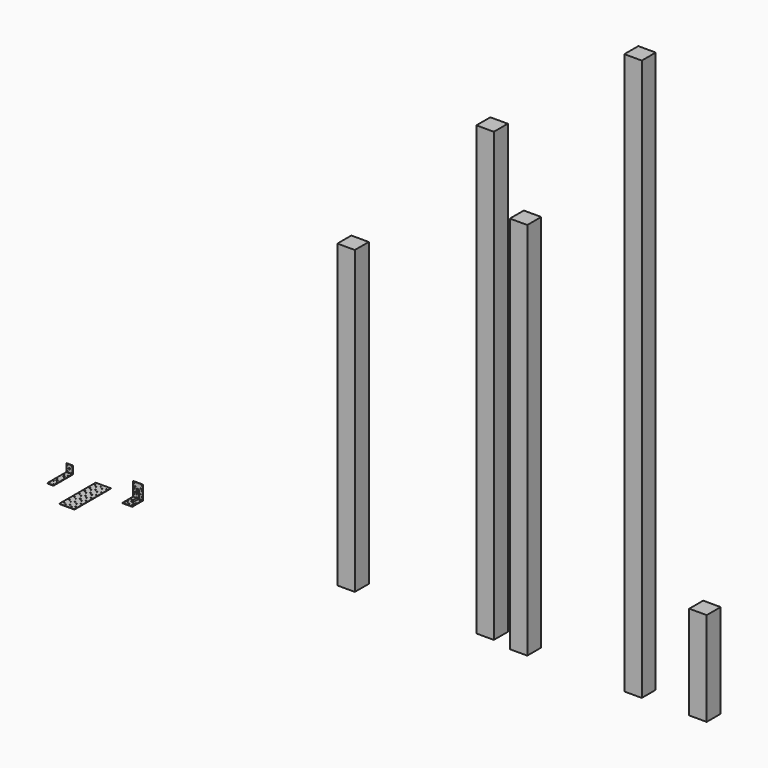
from build123d import *

# Parameters (mm, degrees)
F0_W      = 115
F0_H      = 115
F1_DEPTH  = 1985
F2_W      = 115
F2_H      = 115
F3_DEPTH  = 2950
F4_W      = 115
F4_H      = 115
F5_DEPTH  = 2500
F6_W      = 115
F6_H      = 115
F7_DEPTH  = 3700
F8_W      = 115
F8_H      = 115
F9_DEPTH  = 620
F10_W     = 65
F10_H     = 90
F10_R     = 2.5
F10_R_2   = 4
F11_DEPTH = 2.5
F12_W     = 65
F12_H     = 2.5
F13_DEPTH = 90
F14_W     = 7
F14_H     = 49.849742502
F15_DEPTH = 5
F16_W     = 14
F16_H     = 50
F17_DEPTH = 5
F18_F1_R  = 5
F18_F2_R  = 4.9999
F16_R     = 2.5
F19_DEPTH = 25
F20_W     = 100
F20_H     = 300
F20_R     = 3
F21_DEPTH = 2
F22_W     = 40
F22_H     = 160
F23_DEPTH = 3
F24_W     = 40
F24_H     = 3
F25_DEPTH = 50
F26_R     = 5
F26_R_2   = 2.5
F27_DEPTH = 25
F28_R     = 2
F29_R     = 2.5
F29_R_2   = 5
F30_DEPTH = 25


# Not quite as in the source:
# - a fillet or chamfer is up to 0.001 mm smaller than in the source, because OpenCascade refuses the exact size


with BuildPart() as f1:
    # F0 (on Top) → F1 (new body)
    with BuildSketch(Plane.XY):
        with Locations((-57.5, -57.5)):
            Rectangle(F0_W, F0_H)
    extrude(amount=F1_DEPTH)


with BuildPart() as f3:
    # F2 (on Top) → F3 (new body)
    with BuildSketch(Plane.XY):
        with Locations((835.767865181, -28.2673428646)):
            Rectangle(F2_W, F2_H)
    extrude(amount=F3_DEPTH)


with BuildPart() as f5:
    # F4 (on Top) → F5 (new body)
    with BuildSketch(Plane.XY):
        with Locations((1079.8359951153, -57.5)):
            Rectangle(F4_W, F4_H)
    extrude(amount=F5_DEPTH)


with BuildPart() as f7:
    # F6 (on Top) → F7 (new body)
    with BuildSketch(Plane.XY):
        with Locations((1834.8243838341, -57.5)):
            Rectangle(F6_W, F6_H)
    extrude(amount=F7_DEPTH)


with BuildPart() as f9:
    # F8 (on Top) → F9 (new body)
    with BuildSketch(Plane.XY):
        with Locations((2262.808675766, -57.5)):
            Rectangle(F8_W, F8_H)
    extrude(amount=F9_DEPTH)


with BuildPart() as f11:
    # F10 (on Top) → F11 (new body)
    with BuildSketch(Plane.XY):
        with Locations((-1520.1824146039, -45)):
            Rectangle(F10_W, F10_H)
        with Locations((-1544.6824146039, -81.6684067249)):
            Circle(F10_R, mode=Mode.SUBTRACT)
        with Locations((-1539.6824146039, -63.6286884546)):
            Circle(F10_R, mode=Mode.SUBTRACT)
        with Locations((-1544.6824146039, -50.4504516721)):
            Circle(F10_R, mode=Mode.SUBTRACT)
        with Locations((-1520.1824146039, -77.8877660632)):
            Circle(F10_R_2, mode=Mode.SUBTRACT)
        with Locations((-1495.6824146039, -81.6684067249)):
            Circle(F10_R, mode=Mode.SUBTRACT)
        with Locations((-1500.6824146039, -63.6286884546)):
            Circle(F10_R, mode=Mode.SUBTRACT)
        with Locations((-1495.6824146039, -50.4504516721)):
            Circle(F10_R, mode=Mode.SUBTRACT)
        with Locations((-1539.6824146039, -30.1858838648)):
            Circle(F10_R, mode=Mode.SUBTRACT)
        with Locations((-1544.6824146039, -15.9201901406)):
            Circle(F10_R, mode=Mode.SUBTRACT)
        with Locations((-1500.6824146039, -30.1858838648)):
            Circle(F10_R, mode=Mode.SUBTRACT)
        with Locations((-1495.6824146039, -15.9201901406)):
            Circle(F10_R, mode=Mode.SUBTRACT)
    extrude(amount=F11_DEPTH)

    # F12 (on face) → F13 (join)
    with BuildSketch(Plane.XY.offset(2.5)):
        with Locations((-1520.1824146039, -1.25)):
            Rectangle(F12_W, F12_H)
    extrude(amount=F13_DEPTH)

    # F14 (on face) → F15 (join)
    with BuildSketch(Plane.XY.offset(2.5)):
        with Locations((-1516.6824146039, -27.424871251)):
            Rectangle(F14_W, F14_H)
        with Locations((-1523.6824146039, -27.424871251)):
            Rectangle(F14_W, F14_H)
    extrude(amount=F15_DEPTH)

    # F16 (on face) → F17 (join)
    with BuildSketch(Plane.XZ.offset(2.5)):
        with Locations((-1520.1824146039, 32.5)):
            Rectangle(F16_W, F16_H)
    extrude(amount=F17_DEPTH)

    # F18: fillet of radius 5 on 5 edges, made by hand

    # F18_f1
    f18_f1_edges = [f11.edges().sort_by_distance(p)[0] for p in [
        (-1520.1824146039, -7.5, 7.5),
    ]]
    fillet(f18_f1_edges, radius=F18_F1_R)

    # F18_f2 (radius 5 in the source; OpenCascade refuses exactly that, so slightly less here)
    f18_f2_edges = [f11.edges().sort_by_distance(p)[0] for p in [
        (-1527.1824146039, -32.424871251, 7.5),
        (-1513.1824146039, -7.5, 35),
        (-1520.1824146039, -52.349742502, 7.5),
        (-1520.1824146039, -7.5, 57.5),
        (-1513.1824146039, -8.9644660941, 8.9644660941),
        (-1527.1824146039, -8.9644660941, 8.9644660941),
    ]]
    fillet(f18_f2_edges, radius=F18_F2_R)

    # F16 (on face) → F19 (cut)
    with BuildSketch(Plane.XZ.offset(2.5)):
        with Locations((-1544.6824146039, 18.7368597835)):
            Circle(F16_R)
        with Locations((-1539.6824146039, 33.0025535077)):
            Circle(F16_R)
        with Locations((-1544.6824146039, 53.267121315)):
            Circle(F16_R)
        with Locations((-1539.6824146039, 66.4453580976)):
            Circle(F16_R)
        with Locations((-1544.6824146039, 84.4850763679)):
            Circle(F16_R)
        with Locations((-1495.6824146039, 84.4850763679)):
            Circle(F16_R)
        with Locations((-1500.6824146039, 66.4453580976)):
            Circle(F16_R)
        with Locations((-1495.6824146039, 53.267121315)):
            Circle(F16_R)
        with Locations((-1500.6824146039, 33.0025535077)):
            Circle(F16_R)
        with Locations((-1495.6824146039, 18.7368597835)):
            Circle(F16_R)
    extrude(amount=-F19_DEPTH, mode=Mode.SUBTRACT)


with BuildPart() as f21:
    # F20 (on Top) → F21 (new body)
    with BuildSketch(Plane.XY):
        with Locations((-1750.8230004184, -150)):
            Rectangle(F20_W, F20_H)
        with Locations((-1788.8230004184, -273.6264169216)):
            Circle(F20_R, mode=Mode.SUBTRACT)
        with Locations((-1788.8230004184, -231.6264169216)):
            Circle(F20_R, mode=Mode.SUBTRACT)
        with Locations((-1769.8230004184, -286.8777215481)):
            Circle(F20_R, mode=Mode.SUBTRACT)
        with Locations((-1750.8230004184, -273.6264169216)):
            Circle(F20_R, mode=Mode.SUBTRACT)
        with Locations((-1769.8230004184, -244.8777215481)):
            Circle(F20_R, mode=Mode.SUBTRACT)
        with Locations((-1750.8230004184, -231.6264169216)):
            Circle(F20_R, mode=Mode.SUBTRACT)
        with Locations((-1788.8230004184, -189.6264169216)):
            Circle(F20_R, mode=Mode.SUBTRACT)
        with Locations((-1769.8230004184, -202.8777215481)):
            Circle(F20_R, mode=Mode.SUBTRACT)
        with Locations((-1750.8230004184, -189.6264169216)):
            Circle(F20_R, mode=Mode.SUBTRACT)
        with Locations((-1769.8230004184, -160.8777215481)):
            Circle(F20_R, mode=Mode.SUBTRACT)
        with Locations((-1731.8230004184, -286.8777215481)):
            Circle(F20_R, mode=Mode.SUBTRACT)
        with Locations((-1731.8230004184, -244.8777215481)):
            Circle(F20_R, mode=Mode.SUBTRACT)
        with Locations((-1712.8230004184, -273.6264169216)):
            Circle(F20_R, mode=Mode.SUBTRACT)
        with Locations((-1712.8230004184, -231.6264169216)):
            Circle(F20_R, mode=Mode.SUBTRACT)
        with Locations((-1731.8230004184, -202.8777215481)):
            Circle(F20_R, mode=Mode.SUBTRACT)
        with Locations((-1731.8230004184, -160.8777215481)):
            Circle(F20_R, mode=Mode.SUBTRACT)
        with Locations((-1712.8230004184, -189.6264169216)):
            Circle(F20_R, mode=Mode.SUBTRACT)
        with Locations((-1788.8230004184, -147.6264169216)):
            Circle(F20_R, mode=Mode.SUBTRACT)
        with Locations((-1788.8230004184, -105.6264169216)):
            Circle(F20_R, mode=Mode.SUBTRACT)
        with Locations((-1769.8230004184, -118.8777215481)):
            Circle(F20_R, mode=Mode.SUBTRACT)
        with Locations((-1750.8230004184, -147.6264169216)):
            Circle(F20_R, mode=Mode.SUBTRACT)
        with Locations((-1769.8230004184, -76.8777215481)):
            Circle(F20_R, mode=Mode.SUBTRACT)
        with Locations((-1750.8230004184, -105.6264169216)):
            Circle(F20_R, mode=Mode.SUBTRACT)
        with Locations((-1788.8230004184, -63.6264169216)):
            Circle(F20_R, mode=Mode.SUBTRACT)
        with Locations((-1788.8230004184, -21.6264169216)):
            Circle(F20_R, mode=Mode.SUBTRACT)
        with Locations((-1750.8230004184, -63.6264169216)):
            Circle(F20_R, mode=Mode.SUBTRACT)
        with Locations((-1769.8230004184, -34.8777215481)):
            Circle(F20_R, mode=Mode.SUBTRACT)
        with Locations((-1750.8230004184, -21.6264169216)):
            Circle(F20_R, mode=Mode.SUBTRACT)
        with Locations((-1731.8230004184, -118.8777215481)):
            Circle(F20_R, mode=Mode.SUBTRACT)
        with Locations((-1731.8230004184, -76.8777215481)):
            Circle(F20_R, mode=Mode.SUBTRACT)
        with Locations((-1712.8230004184, -147.6264169216)):
            Circle(F20_R, mode=Mode.SUBTRACT)
        with Locations((-1712.8230004184, -105.6264169216)):
            Circle(F20_R, mode=Mode.SUBTRACT)
        with Locations((-1731.8230004184, -34.8777215481)):
            Circle(F20_R, mode=Mode.SUBTRACT)
        with Locations((-1712.8230004184, -63.6264169216)):
            Circle(F20_R, mode=Mode.SUBTRACT)
        with Locations((-1712.8230004184, -21.6264169216)):
            Circle(F20_R, mode=Mode.SUBTRACT)
    extrude(amount=F21_DEPTH)


with BuildPart() as f23:
    # F22 (on Top) → F23 (new body)
    with BuildSketch(Plane.XY):
        with Locations((-1971.4077202505, -80)):
            Rectangle(F22_W, F22_H)
    extrude(amount=F23_DEPTH)

    # F24 (on face) → F25 (join)
    with BuildSketch(Plane.XY.offset(3)):
        with Locations((-1971.4077202505, -1.5)):
            Rectangle(F24_W, F24_H)
    extrude(amount=F25_DEPTH)

    # F26 (on face) → F27 (cut)
    with BuildSketch(Plane.XZ.offset(3)):
        with Locations((-1971.4077202505, 28)):
            Circle(F26_R)
        with Locations((-1985.5265147915, 10.3515068237)):
            Circle(F26_R_2)
        with Locations((-1985.5265147915, 45.6484931763)):
            Circle(F26_R_2)
        with Locations((-1957.2889257095, 45.6484931763)):
            Circle(F26_R_2)
        with Locations((-1957.2889257095, 10.3515068237)):
            Circle(F26_R_2)
    extrude(amount=-F27_DEPTH, mode=Mode.SUBTRACT)

    # F28
    f28_edges = [f23.edges().sort_by_distance(p)[0] for p in [
        (-1971.40772, -3, 3),
        (-1971.40772, 0, 0),
    ]]
    fillet(f28_edges, radius=F28_R)

    # F29 (on face) → F30 (cut)
    with BuildSketch(Plane.XY.offset(3)):
        with Locations((-1959.4077202505, -30.9613841772)):
            Circle(F29_R)
        with Locations((-1959.4077202505, -60.9613841772)):
            Circle(F29_R)
        with Locations((-1959.4077202505, -90.9613841772)):
            Circle(F29_R)
        with Locations((-1959.4077202505, -120.9613841772)):
            Circle(F29_R)
        with Locations((-1959.4077202505, -150.9613841772)):
            Circle(F29_R)
        with Locations((-1983.4077202505, -150.9613841772)):
            Circle(F29_R)
        with Locations((-1983.4077202505, -120.9613841772)):
            Circle(F29_R)
        with Locations((-1983.4077202505, -90.9613841772)):
            Circle(F29_R)
        with Locations((-1983.4077202505, -60.9613841772)):
            Circle(F29_R)
        with Locations((-1983.4077202505, -30.9613841772)):
            Circle(F29_R)
        with Locations((-1971.4077202505, -47.7219521999)):
            Circle(F29_R_2)
        with Locations((-1971.4077202505, -105.8257073164)):
            Circle(F29_R_2)
    extrude(amount=-F30_DEPTH, mode=Mode.SUBTRACT)


solid = Compound([f1.part, f3.part, f5.part, f7.part, f9.part, f11.part, f21.part, f23.part])
